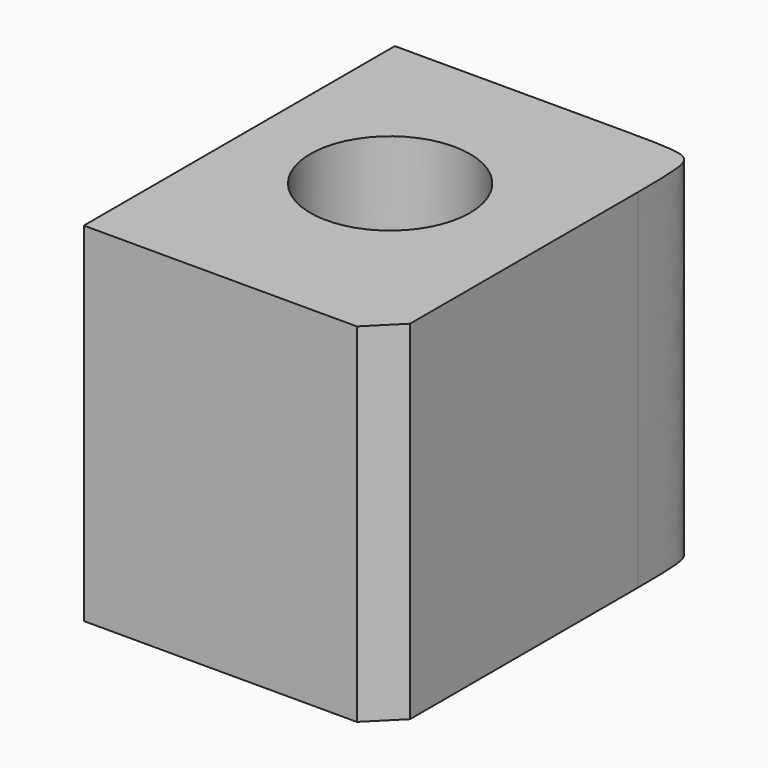
from build123d import *

# Parameters (mm, degrees)
F0_W        = 51.974568516
F0_H        = 66.7630434036
F0_R        = 13.7134635275
F1_DEPTH    = 59.80942
F2_SIZE     = 5.08
F3_T1_DEPTH = 123.30942


# Not quite as in the source:
# - a fillet or chamfer that OpenCascade refuses, or shapes differently, is made with other operations: its cross-section is extruded or revolved along the edge and cut away or added


with BuildPart() as f1:
    # F0 (on Top) → F1 (new body)
    with BuildSketch(Plane.XY):
        with Locations((25.987284258, 33.3815217018)):
            Rectangle(F0_W, F0_H)
        with Locations((24.4355015457, 35.2227129042)):
            Circle(F0_R, mode=Mode.SUBTRACT)
    extrude(amount=F1_DEPTH)

    # F2
    f2_edges = [f1.edges().sort_by_distance(p)[0] for p in [
        (51.974569, 0, 29.90471),
    ]]
    chamfer(f2_edges, length=F2_SIZE)

    # F3: fillet of radius 12.7 on 1 edges, made by hand

    # F3_s2 → F3_t1 (cut)
    with BuildSketch(Plane.XY.offset(-31.75)):
        with BuildLine():
            add(Edge.make_bspline(
                [(51.974568516, 54.0630434036), (51.974568516, 66.7630434036), (39.274568516, 66.7630434036)],
                knots=[0, 0, 0, 1, 1, 1], degree=2, weights=[1, 4, 1]))
            Line((39.274568516, 66.7630434036), (51.974568516, 66.7630434036))
            Line((51.974568516, 66.7630434036), (51.974568516, 54.0630434036))
        make_face()
    extrude(amount=F3_T1_DEPTH, mode=Mode.SUBTRACT)


solid = f1.part
